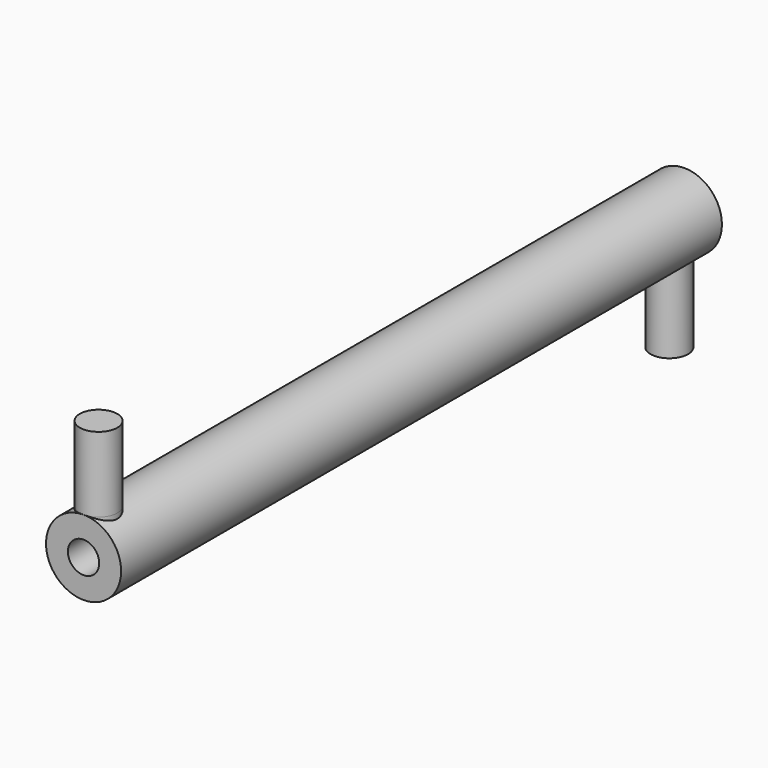
from build123d import *

# Parameters (mm, degrees)
F0_R          = 50
F0_R_2        = 20.8333333333
F1_DEPTH      = 1000
F5_R          = 25
F6_DEPTH      = 100
F6_DEPTH_BACK = 7
F3_R          = 25
F7_DEPTH      = 7
F7_DEPTH_BACK = 100


# Not quite as in the source:
# - a feature names something its author has since deleted; it is built from what else it names


with BuildPart() as f1:
    # F0 (on Front) → F1 (new body)
    with BuildSketch(Plane.XZ):
        Circle(F0_R)
        Circle(F0_R_2, mode=Mode.SUBTRACT)
    extrude(amount=-F1_DEPTH)

    # F5 (on offset) → F6 (join, two sides)
    with BuildSketch(Plane.XY.offset(-50)) as f6_sk:
        with Locations((0, 975)):
            Circle(F5_R)
    extrude(amount=-F6_DEPTH)
    extrude(f6_sk.sketch, amount=F6_DEPTH_BACK)


with BuildPart() as f7:
    # F3 (on offset) → F7 (new body, two sides)
    with BuildSketch(Plane.XY.offset(50)) as f7_sk:
        with Locations((0, 25)):
            Circle(F3_R)
    extrude(amount=-F7_DEPTH)
    extrude(f7_sk.sketch, amount=F7_DEPTH_BACK)


solid = Compound([f1.part, f7.part])
